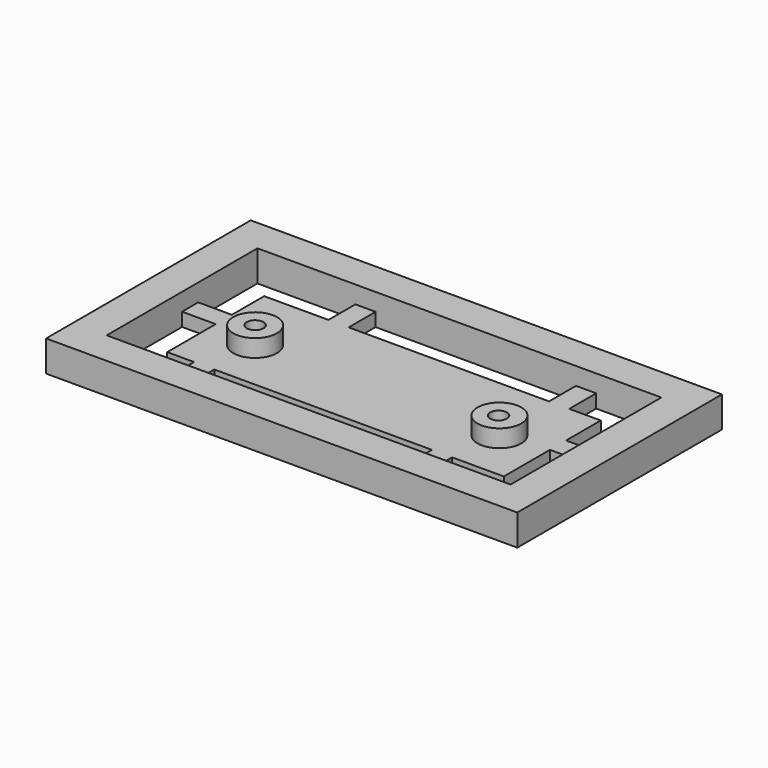
from build123d import *

# Parameters (mm, degrees)
F1_DEPTH  = 2
F2_R      = 3.25
F3_DEPTH  = 2.6
F0_W      = 3
F0_H      = 5
F5_DEPTH  = 2
F6_R      = 1.25
F7_DEPTH  = 25
F8_R      = 1.25
F9_DEPTH  = 25
F0_W_2    = 5
F0_H_2    = 3
F10_DEPTH = 2
F11_DEPTH = 2
F12_DEPTH = 2
F13_DEPTH = 2
F14_W     = 70
F14_H     = 38
F14_W_2   = 60
F14_H_2   = 28
F15_DEPTH = 4.6


# Not quite as in the source:
# - a feature names something its author has since deleted; it is built from what else it names


with BuildPart() as f1:
    # F0 (on Top) → F1 (new body)
    with BuildSketch(Plane.XY):
        Polygon((-13.6037096381, 18), (-23.153355509, 18), (-23.153355509, 12), (-23.153355509, 9), (-23.153355509, 0), (-19.1677454859, 0), (-16.1677454859, 0), (16.1677454859, 0), (19.1677454859, 0), (23.153355509, 0), (26.846644491, 0), (26.846644491, 8.565065451), (26.846644491, 11.565065451), (26.846644491, 18), (22.1654525697, 18), (19.1654525697, 18), (-10.6037096381, 18), align=None)
    extrude(amount=F1_DEPTH)

    # F2 (on face) → F3 (join)
    with BuildSketch(Plane.XY.offset(2)):
        with Locations((19.996644491, 7.75)):
            Circle(F2_R)
        with Locations((-16.303355509, 7.75)):
            Circle(F2_R)
    extrude(amount=F3_DEPTH)

    # F0 (on Top) → F5 (join)
    with BuildSketch(Plane.XY):
        with Locations((20.6654525697, 20.5)):
            Rectangle(F0_W, F0_H)
    extrude(amount=F5_DEPTH)

    # F6 (on face) → F7 (cut)
    with BuildSketch(Plane.XY.offset(4.6)):
        with Locations((-16.303355509, 7.75)):
            Circle(F6_R)
    extrude(amount=-F7_DEPTH, mode=Mode.SUBTRACT)

    # F8 (on face) → F9 (cut)
    with BuildSketch(Plane.XY.offset(4.6)):
        with Locations((19.9292600155, 7.6608564705)):
            Circle(F8_R)
    extrude(amount=-F9_DEPTH, mode=Mode.SUBTRACT)

    # F0 (on Top) → F10 (join)
    with BuildSketch(Plane.XY):
        with Locations((29.346644491, 10.065065451)):
            Rectangle(F0_W_2, F0_H_2)
        with Locations((-25.653355509, 10.5)):
            Rectangle(F0_W_2, F0_H_2)
    extrude(amount=F10_DEPTH)

    # F0 (on Top) → F11 (join)
    with BuildSketch(Plane.XY):
        with Locations((17.6677454859, -2.5)):
            Rectangle(F0_W, F0_H)
    extrude(amount=F11_DEPTH)

    # F0 (on Top) → F12 (join)
    with BuildSketch(Plane.XY):
        with Locations((-17.6677454859, -2.5)):
            Rectangle(F0_W, F0_H)
    extrude(amount=F12_DEPTH)

    # F0 (on Top) → F13 (join)
    with BuildSketch(Plane.XY):
        with Locations((-12.1037096381, 20.5)):
            Rectangle(F0_W, F0_H)
    extrude(amount=F13_DEPTH)

    # F14 (on Top) → F15 (join)
    with BuildSketch(Plane.XY):
        with Locations((1.846644491, 9)):
            Rectangle(F14_W, F14_H)
        with Locations((1.846644491, 9)):
            Rectangle(F14_W_2, F14_H_2, mode=Mode.SUBTRACT)
    extrude(amount=F15_DEPTH)


solid = f1.part
